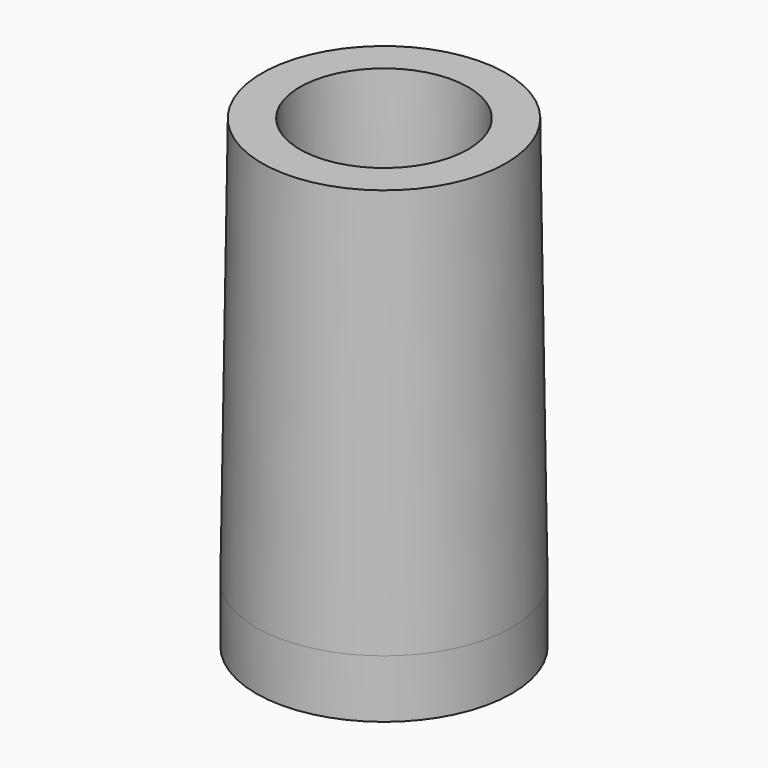
from build123d import *

# Parameters (mm, degrees)
F0_R     = 11
F0_R_2   = 6.75
F1_DEPTH = 40
F0_R_3   = 4
F2_DEPTH = 20
F3_SIZE2 = 19.99999
F3_SIZE  = 0.49999
F4_SIZE2 = 35
F4_SIZE  = 0.5


# Not quite as in the source:
# - a fillet or chamfer is up to 0.001 mm smaller than in the source, because OpenCascade refuses the exact size


with BuildPart() as f1:
    # F0 (on Top) → F1 (new body)
    with BuildSketch(Plane.XY):
        Circle(F0_R)
        Circle(F0_R_2, mode=Mode.SUBTRACT)
    extrude(amount=F1_DEPTH)

    # F0 (on Top) → F2 (join)
    with BuildSketch(Plane.XY):
        Circle(F0_R_2)
        Circle(F0_R_3, mode=Mode.SUBTRACT)
    extrude(amount=F2_DEPTH)

    # F3 (size 0.5 and 20 in the source; OpenCascade refuses exactly that, so slightly less here)
    f3_edges = [f1.edges().sort_by_distance(p)[0] for p in [
        (-6.75, 0, 40),
    ]]
    f3_side = f1.faces().sort_by_distance((-10.688873, 0, 40))[0]
    chamfer(f3_edges, length=F3_SIZE, length2=F3_SIZE2, reference=f3_side)

    # F4
    f4_edges = [f1.edges().sort_by_distance(p)[0] for p in [
        (-11, 0, 40),
    ]]
    f4_side = f1.faces().sort_by_distance((-7.561117, 0, 40))[0]
    chamfer(f4_edges, length=F4_SIZE, length2=F4_SIZE2, reference=f4_side)


solid = f1.part
